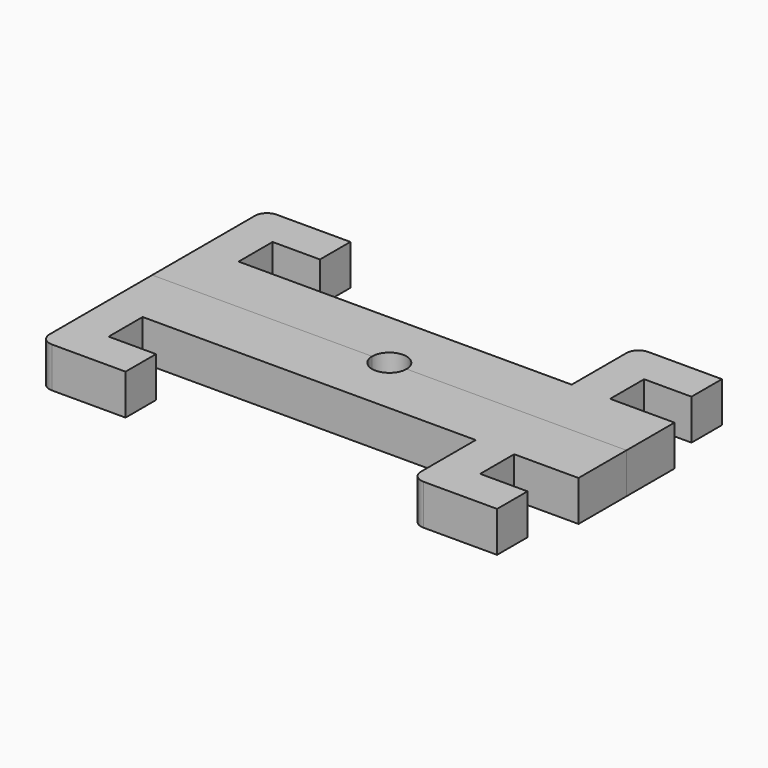
from build123d import *
from build123d import SkipClean  # not in build123d's __all__

# Parameters (mm, degrees)
F1_DEPTH = 5
F2_R     = 1.5


with BuildPart() as f1:
    # F0 (on Top) → F1 (new body)
    with BuildSketch(Plane.XY):
        with BuildLine():
            ThreePointArc((-2.125, 0), (0, 2.125), (2.125, 0))
            Line((2.125, 0), (29.3, 0))
            Line((29.3, 0), (29.3, 7.41))
            Line((29.3, 7.41), (21.35, 7.41))
            Line((21.35, 7.41), (21.35, 12.66))
            Line((21.35, 12.66), (27.2, 12.66))
            Line((27.2, 12.66), (27.2, 17.36))
            Line((27.2, 17.36), (16.6, 17.36))
            Line((16.6, 17.36), (16.6, 7.41))
            Line((16.6, 7.41), (-24.55, 7.41))
            Line((-24.55, 7.41), (-24.55, 12.66))
            Line((-24.55, 12.66), (-18.7, 12.66))
            Line((-18.7, 12.66), (-18.7, 17.36))
            Line((-18.7, 17.36), (-29.3, 17.36))
            Line((-29.3, 17.36), (-29.3, 0))
            Line((-29.3, 0), (-2.125, 0))
        make_face()
    extrude(amount=F1_DEPTH)

    # F2
    f2_edges = [f1.edges().sort_by_distance(p)[0] for p in [
        (-29.3, 17.36, 2.5),
        (16.6, 17.36, 2.5),
    ]]
    fillet(f2_edges, radius=F2_R)

    # F3: F1 across face


with BuildPart() as f1_1:
    add(f1.part, clean=False)
    with SkipClean():  # cleaning this boolean's faces spoils the solid; the shape is the same uncleaned
        add(f1.part.mirror(Plane(origin=(-15.7125, 0, 2.5), x_dir=(1, 0, 0), z_dir=(0, -1, 0))), clean=False)


solid = f1_1.part
